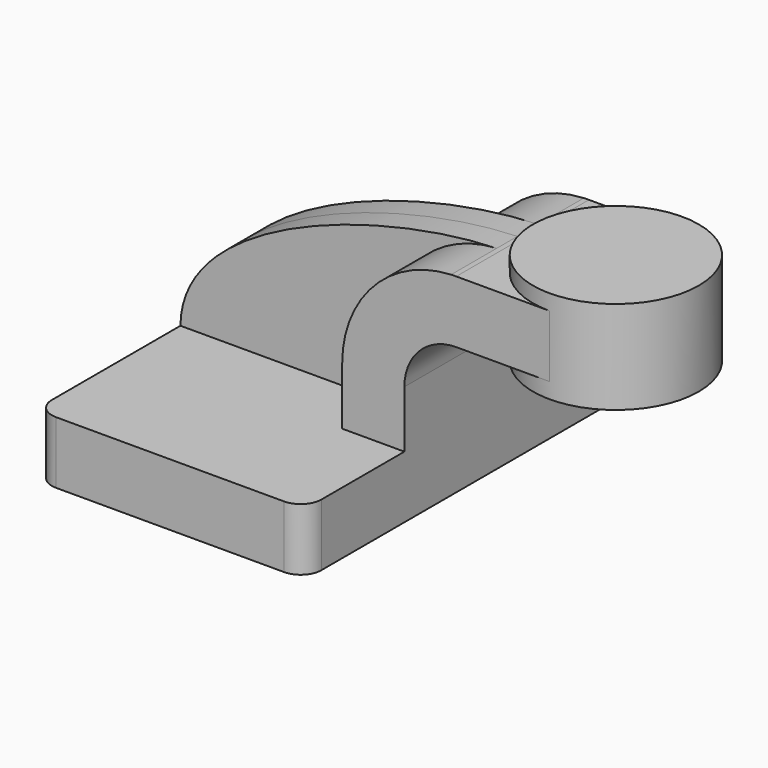
from build123d import *

# Parameters (mm, degrees)
F1_DEPTH = 63.5
F0_W     = 25.4
F0_H     = 19.0499988828
F2_DEPTH = 25.4
F3_DEPTH = 7.9375
F5_R     = 6.35


# Not quite as in the source:
# - ends of sketch curves that miss each other by under 0.0002 mm in the source are joined


with BuildPart() as f1:
    # F0 (on Front) → F1 (new body, symmetric)
    with BuildSketch(Plane.XZ):
        Polygon((41.275, -9.525), (41.275, 9.525), (22.2249999642, 9.525), (-41.275, 9.525), (-41.275, -9.525), align=None)
    extrude(amount=F1_DEPTH, both=True)

    # F0 (on Front) → F2 (join, symmetric)
    with BuildSketch(Plane.XZ):
        with Locations((73.025, 52.4001994414)):
            Rectangle(F0_W, F0_H)
        with BuildLine():
            Line((22.2249999642, 9.525), (41.275, 9.525))
            Line((41.275, 9.525), (41.275, 27.0002))
            ThreePointArc((41.275, 27.0002), (45.9246798487, 38.2255201513), (57.15, 42.8752))
            Line((57.15, 42.8752), (60.325, 42.8752))
            Line((60.325, 42.8752), (60.325, 61.9251988828))
            Line((60.325, 61.9251988828), (57.15, 61.9251988828))
            add(Edge.make_bspline(
                [(55.577466475, 61.8897796164), (56.107456948, 61.9056705872), (56.6317308349, 61.9174837091), (57.15, 61.9251988828)],
                knots=[109.8639655387, 109.8639655387, 109.8639655387, 109.8639655387, 111.5045361803, 111.5045361803, 111.5045361803, 111.5045361803], degree=3))
            ThreePointArc((55.577466475, 61.8897796164), (31.9044423619, 51.133526481), (22.2249999642, 27.0002))
            Line((22.2249999642, 27.0002), (22.2249999642, 9.525))
        make_face()
    extrude(amount=F2_DEPTH, both=True)

    # F0 (on Front) → F3 (join, symmetric)
    with BuildSketch(Plane.XZ):
        with BuildLine():
            Line((-41.275, 9.525), (22.2249999642, 9.525))
            Line((22.2249999642, 9.525), (22.2249999642, 27.0002))
            ThreePointArc((22.2249999642, 27.0002), (31.9044423619, 51.133526481), (55.577466475, 61.8897796164))
            add(Edge.make_bspline(
                [(-41.275, 9.525), (-41.042616605, 41.4740477998), (20.0856360221, 60.8256102231), (55.577466475, 61.8897796164)],
                knots=[0, 0, 0, 0, 109.8639655387, 109.8639655387, 109.8639655387, 109.8639655387], degree=3))
        make_face()
    extrude(amount=F3_DEPTH, both=True)

    # F0 (on Front) → F4 (revolve)
    with BuildSketch(Plane.XZ):
        Polygon((85.725, 61.9251988828), (85.725, 42.8752), (85.725, 38.1), (111.125, 38.1), (111.125, 66.675), (85.725, 66.675), align=None)
    revolve(axis=Axis((85.725, 0, 52.3875), (0, 0, 1)))

    # F5
    f5_edges = [f1.edges().sort_by_distance(p)[0] for p in [
        (41.275, -63.5, 0),
        (41.275, 63.5, 0),
        (-41.275, -63.5, 0),
        (-41.275, 63.5, 0),
    ]]
    fillet(f5_edges, radius=F5_R)


solid = f1.part
